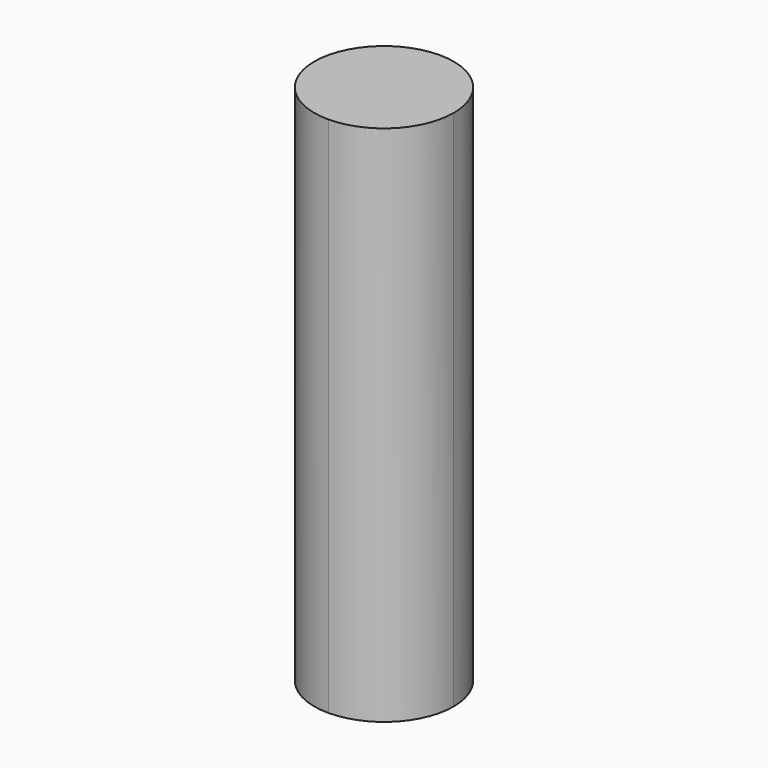
from build123d import *

# Parameters (mm, degrees)
F0_W     = 10.16
F0_H     = 38.1
F1_DEPTH = 10.16
F2_R     = 5.07999


# Not quite as in the source:
# - a fillet or chamfer is up to 0.001 mm smaller than in the source, because OpenCascade refuses the exact size


with BuildPart() as f1:
    # F0 (on Front) → F1 (new body)
    with BuildSketch(Plane.XZ):
        with Locations((-0.8241977656, -2.1479204297)):
            Rectangle(F0_W, F0_H)
    extrude(amount=F1_DEPTH)

    # F2 (radius 5.08 in the source; OpenCascade refuses exactly that, so slightly less here)
    f2_edges = [f1.edges().sort_by_distance(p)[0] for p in [
        (4.255802, -10.16, -2.14792),
        (-5.904198, -10.16, -2.14792),
        (-5.904198, 0, -2.14792),
        (4.255802, 0, -2.14792),
    ]]
    fillet(f2_edges, radius=F2_R)


solid = f1.part
